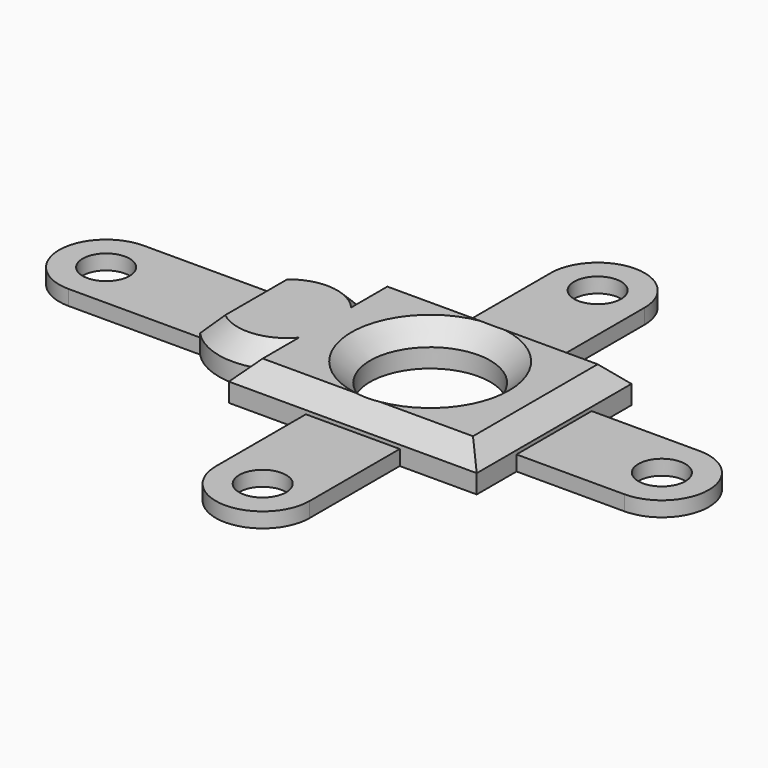
from build123d import *

# Parameters (mm, degrees)
F0_R         = 4.064
F1_DEPTH     = 2.54
F0_R_2       = 1.5875
F2_DEPTH     = 1.016
F3_T1_DEPTH  = 23.2960747894
F3_T3_DEPTH  = 19.6130747894
F3_T5_DEPTH  = 12.8820747894
F3_T10_DEPTH = 8.6144406225
F3_S11_R     = 4.6355
F3_T12_DEPTH = 6
F3_T16_ANGLE = 143.4241535748
F3_T21_ANGLE = 143.4241535748
F3_T26_DEPTH = 8.6144406225
F3_S27_R     = 4.6355
F3_T28_DEPTH = 6
F3_T35_ANGLE = 143.4241535748
F3_T39_DEPTH = 8.6144406225
F3_S40_R     = 4.6355
F3_T41_DEPTH = 6
F3_T47_DEPTH = 8.6144406225
F3_S48_R     = 4.6355
F3_T49_DEPTH = 6
F3_T52_ANGLE = 143.4241535748


# Not quite as in the source:
# - a fillet or chamfer that OpenCascade refuses, or shapes differently, is made with other operations: its cross-section is extruded or revolved along the edge and cut away or added
# - a feature names something its author has since deleted; it is built from what else it names


with BuildPart() as f1:
    # F0 (on Top) → F1 (new body)
    with BuildSketch(Plane.XY):
        Polygon((-8.382, 6.5405), (-8.382, 4.4581341669), (-8.382, -4.4581341669), (-8.382, -6.5405), (-3.175, -6.5405), (3.175, -6.5405), (8.382, -6.5405), (8.382, -3.175), (8.382, 3.175), (8.382, 6.5405), (3.175, 6.5405), (-3.175, 6.5405), align=None)
        Circle(F0_R, mode=Mode.SUBTRACT)
        with BuildLine():
            Line((-8.382, -4.4581341669), (-8.382, 4.4581341669))
            ThreePointArc((-8.382, 4.4581341669), (-10.8856754478, 4.4683224077), (-13.0294598813, 3.175))
            Line((-13.0294598813, 3.175), (-13.0294598813, -3.175))
            ThreePointArc((-13.0294598813, -3.175), (-10.8856754478, -4.4683224077), (-8.382, -4.4581341669))
        make_face()
    extrude(amount=F1_DEPTH)

    # F0 (on Top) → F2 (join)
    with BuildSketch(Plane.XY):
        with BuildLine():
            Line((-13.0294598813, -3.175), (-13.0294598813, 3.175))
            Line((-13.0294598813, 3.175), (-21.9194598813, 3.175))
            ThreePointArc((-21.9194598813, 3.175), (-25.0944598813, 0), (-21.9194598813, -3.175))
            Line((-21.9194598813, -3.175), (-13.0294598813, -3.175))
        make_face()
        with Locations((-21.9194598813, 0)):
            Circle(F0_R_2, mode=Mode.SUBTRACT)
        with BuildLine():
            Line((3.175, -6.5405), (-3.175, -6.5405))
            Line((-3.175, -6.5405), (-3.175, -14.1605))
            ThreePointArc((-3.175, -14.1605), (0, -17.3355), (3.175, -14.1605))
            Line((3.175, -14.1605), (3.175, -6.5405))
        make_face()
        with Locations((0, -14.1605)):
            Circle(F0_R_2, mode=Mode.SUBTRACT)
        with BuildLine():
            Line((-3.175, 14.1605), (-3.175, 6.5405))
            Line((-3.175, 6.5405), (3.175, 6.5405))
            Line((3.175, 6.5405), (3.175, 14.1605))
            ThreePointArc((3.175, 14.1605), (0, 17.3355), (-3.175, 14.1605))
        make_face()
        with Locations((0, 14.1605)):
            Circle(F0_R_2, mode=Mode.SUBTRACT)
        with BuildLine():
            Line((15.6725401187, 3.175), (8.382, 3.175))
            Line((8.382, 3.175), (8.382, -3.175))
            Line((8.382, -3.175), (15.6725401187, -3.175))
            ThreePointArc((15.6725401187, -3.175), (18.8475401187, 0), (15.6725401187, 3.175))
        make_face()
        with Locations((15.6725401187, 0)):
            Circle(F0_R_2, mode=Mode.SUBTRACT)
    extrude(amount=F2_DEPTH)

    # F3: chamfer of 1.27 on 9 edges, made by hand

    # F3_s2 → F3_t1 (cut)
    with BuildSketch(Plane.YZ.offset(-11.6480373947)):
        Polygon((-5.2705, 2.54), (-6.5405, 1.27), (-6.5405, 2.54), align=None)
        Polygon((6.5405, 1.27), (5.2705, 2.54), (6.5405, 2.54), align=None)
    extrude(amount=F3_T1_DEPTH, mode=Mode.SUBTRACT)

    # F3_s4 → F3_t3 (cut)
    with BuildSketch(Plane.XZ.offset(-9.8065373947)):
        Polygon((7.112, 2.54), (8.382, 1.27), (8.382, 2.54), align=None)
    extrude(amount=F3_T3_DEPTH, mode=Mode.SUBTRACT)

    # F3_s6 → F3_t5 (cut)
    with BuildSketch(Plane.XZ.offset(-6.4410373947)):
        Polygon((-11.7594598813, 2.54), (-13.0294598813, 1.27), (-13.0294598813, 2.54), align=None)
    extrude(amount=F3_T5_DEPTH, mode=Mode.SUBTRACT)


with BuildPart() as f3_tool8:
    # F3_s9 → F3_t10 (new body)
    with BuildSketch(Plane.XZ.offset(1.1920967722)):
        Polygon((-7.112, 2.54), (-8.382, 1.27), (-8.382, 2.54), align=None)
    extrude(amount=F3_T10_DEPTH)

    # F3_s11 → F3_t12 (cut, symmetric)
    with BuildSketch(Plane.XY.offset(1.9)):
        with Locations((-9.652, 0)):
            Circle(F3_S11_R)
    extrude(amount=F3_T12_DEPTH, both=True, mode=Mode.SUBTRACT)


with BuildPart() as f1_1:
    add(f1.part)

    # F3_t7: cut F3_tool8
    add(f3_tool8.part, mode=Mode.SUBTRACT)


with BuildPart() as f3_tool14:
    # F3_s15 → F3_t16 (revolve)
    with BuildSketch(Plane(origin=(-0.0239192805, 0.47989245, 0), x_dir=(0, 0, 1), z_dir=(-0.0497812044, 0.9987601472, 0))):
        Polygon((2.54, -13.005532941), (1.27, -14.275532941), (2.54, -14.275532941), align=None)
    revolve(axis=Axis((-9.652, 0, 2.54), (0, 0, 1)), revolution_arc=F3_T16_ANGLE)

    split(bisect_by=Plane.YZ.offset(-8.382), keep=Keep.BOTTOM)


with BuildPart() as f1_2:
    add(f1_1.part)

    # F3_t13: cut F3_tool14
    add(f3_tool14.part, mode=Mode.SUBTRACT)


with BuildPart() as f3_tool19:
    # F3_s20 → F3_t21 (revolve)
    with BuildSketch(Plane(origin=(-2.9748772597, 4.4568621922, 0), x_dir=(0, 0, 1), z_dir=(0.5551698459, -0.831737003, 0))):
        Polygon((1.27, 3.3924255533), (2.54, 4.6624255533), (2.54, 3.3924255533), align=None)
    revolve(axis=Axis((-9.652, 0, 2.54), (0, 0, 1)), revolution_arc=F3_T21_ANGLE)

    split(bisect_by=Plane.YZ.offset(-8.382), keep=Keep.BOTTOM)


with BuildPart() as f1_3:
    add(f1_2.part)

    # F3_t18: cut F3_tool19
    add(f3_tool19.part, mode=Mode.SUBTRACT)


with BuildPart() as f3_tool24:
    # F3_s25 → F3_t26 (new body)
    with BuildSketch(Plane.XZ.offset(-9.8065373947)):
        Polygon((-8.382, 1.27), (-7.112, 2.54), (-8.382, 2.54), align=None)
    extrude(amount=F3_T26_DEPTH)

    # F3_s27 → F3_t28 (cut, symmetric)
    with BuildSketch(Plane.XY.offset(1.9)):
        with Locations((-9.652, 0)):
            Circle(F3_S27_R)
    extrude(amount=F3_T28_DEPTH, both=True, mode=Mode.SUBTRACT)


with BuildPart() as f1_4:
    add(f1_3.part)

    # F3_t23: cut F3_tool24
    add(f3_tool24.part, mode=Mode.SUBTRACT)

    # F3_s29 → F3_t30 (revolve, cut)
    with BuildSketch(Plane.XZ):
        Polygon((5.334, 2.54), (4.064, 1.27), (4.064, 2.54), align=None)
    revolve(axis=Axis((0, 0, 2.54), (0, 0, 1)), mode=Mode.SUBTRACT)


with BuildPart() as f3_tool33:
    # F3_s34 → F3_t35 (revolve)
    with BuildSketch(Plane(origin=(-0.0239192805, 0.47989245, 0), x_dir=(0, 0, 1), z_dir=(-0.0497812044, 0.9987601472, 0))):
        Polygon((2.54, -13.005532941), (1.27, -14.275532941), (2.54, -14.275532941), align=None)
    revolve(axis=Axis((-9.652, 0, 2.54), (0, 0, 1)), revolution_arc=F3_T35_ANGLE)

    split(bisect_by=Plane.YZ.offset(-8.382), keep=Keep.TOP)


with BuildPart() as f3_tool37:
    # F3_s38 → F3_t39 (new body)
    with BuildSketch(Plane.XZ.offset(1.1920967722)):
        Polygon((-7.112, 2.54), (-8.382, 1.27), (-8.382, 2.54), align=None)
    extrude(amount=F3_T39_DEPTH)

    # F3_s40 → F3_t41 (intersect, symmetric)
    with BuildSketch(Plane.XY.offset(1.9)):
        with Locations((-9.652, 0)):
            Circle(F3_S40_R)
    extrude(amount=F3_T41_DEPTH, both=True, mode=Mode.INTERSECT)


with BuildPart() as f3_tool33_1:
    add(f3_tool33.part)

    # F3_t42: intersect F3_tool37
    add(f3_tool37.part, mode=Mode.INTERSECT)


with BuildPart() as f1_5:
    add(f1_4.part)

    # F3_t31: cut F3_tool33
    add(f3_tool33_1.part, mode=Mode.SUBTRACT)


with BuildPart() as f3_tool45:
    # F3_s46 → F3_t47 (new body)
    with BuildSketch(Plane.XZ.offset(-9.8065373947)):
        Polygon((-8.382, 1.27), (-7.112, 2.54), (-8.382, 2.54), align=None)
    extrude(amount=F3_T47_DEPTH)

    # F3_s48 → F3_t49 (intersect, symmetric)
    with BuildSketch(Plane.XY.offset(1.9)):
        with Locations((-9.652, 0)):
            Circle(F3_S48_R)
    extrude(amount=F3_T49_DEPTH, both=True, mode=Mode.INTERSECT)


with BuildPart() as f3_tool50:
    # F3_s51 → F3_t52 (revolve)
    with BuildSketch(Plane(origin=(-2.9748772597, 4.4568621922, 0), x_dir=(0, 0, 1), z_dir=(0.5551698459, -0.831737003, 0))):
        Polygon((1.27, 3.3924255533), (2.54, 4.6624255533), (2.54, 3.3924255533), align=None)
    revolve(axis=Axis((-9.652, 0, 2.54), (0, 0, 1)), revolution_arc=F3_T52_ANGLE)

    split(bisect_by=Plane.YZ.offset(-8.382), keep=Keep.TOP)


with BuildPart() as f3_tool45_1:
    add(f3_tool45.part)

    # F3_t54: intersect F3_tool50
    add(f3_tool50.part, mode=Mode.INTERSECT)


with BuildPart() as f1_6:
    add(f1_5.part)

    # F3_t43: cut F3_tool45
    add(f3_tool45_1.part, mode=Mode.SUBTRACT)


solid = f1_6.part
